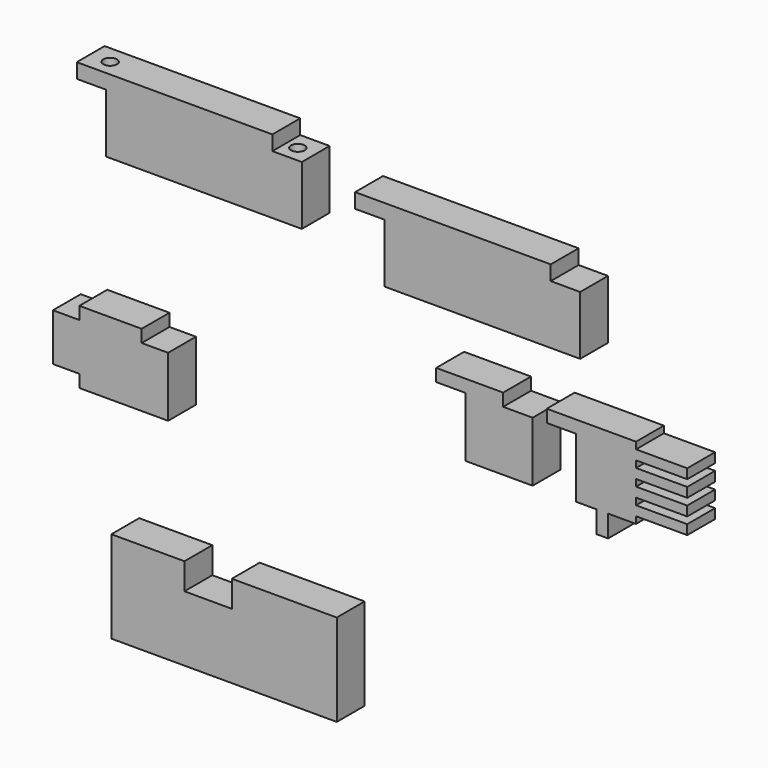
from build123d import *

# Parameters (mm, degrees)
F0_W     = 10.7435509562
F0_H     = 5.3717717528
F0_H_2   = 17.2664299607
F0_H_3   = 4.2206794024
F1_DEPTH = 12.7
F2_DEPTH = 12.7
F0_W_2   = 9.654417634
F0_H_4   = 17.272
F0_W_3   = 9.652
F0_H_5   = 4.572
F3_DEPTH = 12.7
F4_DEPTH = 12.7
F5_R     = 2.4765
F6_DEPTH = 181.0494751265
F0_W_4   = 10.7442
F7_DEPTH = 12.7
F0_W_5   = 4.259288311
F0_H_6   = 7.9820062965
F0_W_6   = 18.6839207555
F0_H_7   = 3.5167981537
F8_DEPTH = 12.7


# Not quite as in the source:
# - a feature names something its author has since deleted; it is built from what else it names


with BuildPart() as f1:
    # F0 (on Front) → F1 (new body)
    with BuildSketch(Plane.XZ):
        Polygon((60.4302587326, 91.194928045), (-0.1946078347, 91.194928045), (-0.1946078347, 85.8231562922), (-0.1946078347, 68.5567263315), (-0.1946078347, 64.3360469291), (60.4302587326, 64.3360469291), (60.4302587326, 68.5567263315), (60.4302587326, 85.8231562922), align=None)
        with Locations((-5.5663833129, 88.5090421686)):
            Rectangle(F0_W, F0_H)
        with Locations((65.8020342107, 77.1899413118)):
            Rectangle(F0_W, F0_H_2)
        with Locations((65.8020342107, 66.4463866303)):
            Rectangle(F0_W, F0_H_3)
    extrude(amount=F1_DEPTH)


with BuildPart() as f2:
    # F0 (on Front) → F2 (new body)
    with BuildSketch(Plane.XZ):
        Polygon((-73.2007697225, -47.6094222765), (-99.8716428876, -47.6094222765), (-99.8716428876, -81.1416803997), (-17.6227167249, -81.1416803997), (-17.6227167249, -47.6094222765), (-55.9287697225, -47.6094222765), (-55.9287697225, -57.2614222765), (-73.2007697225, -57.2614222765), align=None)
    extrude(amount=F2_DEPTH)


with BuildPart() as f3:
    # F0 (on Front) → F3 (new body)
    with BuildSketch(Plane.XZ):
        Polygon((-88.8206250172, 21.9615809619), (-111.5369013648, 21.9615809619), (-111.5369013648, 17.3979116636), (-111.5369013648, 0.1259116636), (-111.5369013648, -4.4460883364), (-88.8206250172, -4.4460883364), (-88.8206250172, 0.1259116636), (-88.8206250172, 17.3979116636), align=None)
        with Locations((-83.9934162002, 8.7619116636)):
            Rectangle(F0_W_2, F0_H_4)
        with Locations((-116.3629013648, 8.7619116636)):
            Rectangle(F0_W_3, F0_H_4)
        with Locations((-83.9934162002, -2.1600883364)):
            Rectangle(F0_W_2, F0_H_5)
    extrude(amount=F3_DEPTH)


with BuildPart() as f4:
    # F0 (on Front) → F4 (new body)
    with BuildSketch(Plane.XZ):
        with Locations((-107.1205325425, 97.2209088504)):
            Rectangle(F0_W, F0_H)
        Polygon((-41.1243997514, 99.9067947268), (-101.7487570643, 99.9067947268), (-101.7487570643, 94.535022974), (-101.7487570643, 77.2685930133), (-101.7487570643, 73.0479136109), (-41.1243997514, 73.0479136109), (-41.1243997514, 77.2685930133), (-41.1243997514, 94.535022974), align=None)
        with Locations((-35.7526242733, 85.9018079937)):
            Rectangle(F0_W, F0_H_2)
        with Locations((-35.7526242733, 75.1582533121)):
            Rectangle(F0_W, F0_H_3)
    extrude(amount=F4_DEPTH)

    # F5 (on face) → F6 (cut, through all)
    with BuildSketch(Plane.XY.offset(99.9067947268)):
        with Locations((-105.1898080206, -6.5809087828)):
            Circle(F5_R)
        with Locations((-36.7368080206, -6.5809087828)):
            Circle(F5_R)
    extrude(amount=-F6_DEPTH, mode=Mode.SUBTRACT)


with BuildPart() as f7:
    # F0 (on Front) → F7 (new body)
    with BuildSketch(Plane.XZ):
        Polygon((43.0781543255, 44.3685778238), (29.4023611633, 44.3685778238), (29.4023611633, 39.7965778238), (29.4023611633, 22.5245778238), (29.4023611633, 17.9525778238), (43.0781543255, 17.9525778238), (43.0781543255, 22.5245778238), (43.0781543255, 39.7965778238), align=None)
        with Locations((24.0302611633, 42.0825778238)):
            Rectangle(F0_W_4, F0_H_5)
        with Locations((48.4502543255, 31.1605778238)):
            Rectangle(F0_W_4, F0_H_4)
        with Locations((48.4502543255, 20.2385778238)):
            Rectangle(F0_W_4, F0_H_5)
    extrude(amount=F7_DEPTH)


with BuildPart() as f8:
    # F0 (on Front) → F8 (new body)
    with BuildSketch(Plane.XZ):
        Polygon((69.7237410633, 44.3685778238), (69.7237410633, 39.7965778238), (69.7237410633, 22.5245778238), (69.7237410633, 17.9525778238), (77.106536278, 17.9525778238), (81.365824589, 17.9525778238), (91.5455787269, 17.9525778238), (91.5455787269, 19.9959375066), (91.5455787269, 20.4223393008), (91.5455787269, 23.6873332513), (91.5455787269, 23.9391374546), (91.5455787269, 26.4088989316), (91.5455787269, 28.5145420683), (91.5455787269, 29.9256970853), (91.5455787269, 32.205937813), (91.5455787269, 32.3954585623), (91.5455787269, 35.9122567161), (91.5455787269, 38.106836158), (91.5455787269, 38.3820181931), (91.5455787269, 41.8988163468), (91.5455787269, 44.3685778238), align=None)
        with Locations((79.2361804335, 13.9615746756)):
            Rectangle(F0_W_5, F0_H_6)
        with Locations((100.8875391047, 40.14041727)):
            Rectangle(F0_W_6, F0_H_7)
        with Locations((100.8875391047, 34.1538576392)):
            Rectangle(F0_W_6, F0_H_7)
        Polygon((110.2294994825, 29.9256970853), (91.5455787269, 29.9256970853), (91.5455787269, 28.5145420683), (91.5455787269, 26.4088989316), (110.2294994825, 26.4088989316), align=None)
        Polygon((91.5455787269, 23.6873332513), (91.5455787269, 20.4223393008), (110.2294994825, 20.4223393008), (110.2294994825, 23.9391374546), (91.5455787269, 23.9391374546), align=None)
        with Locations((64.3516410633, 42.0825778238)):
            Rectangle(F0_W_4, F0_H_5)
    extrude(amount=F8_DEPTH)


solid = Compound([f1.part, f2.part, f3.part, f4.part, f7.part, f8.part])
